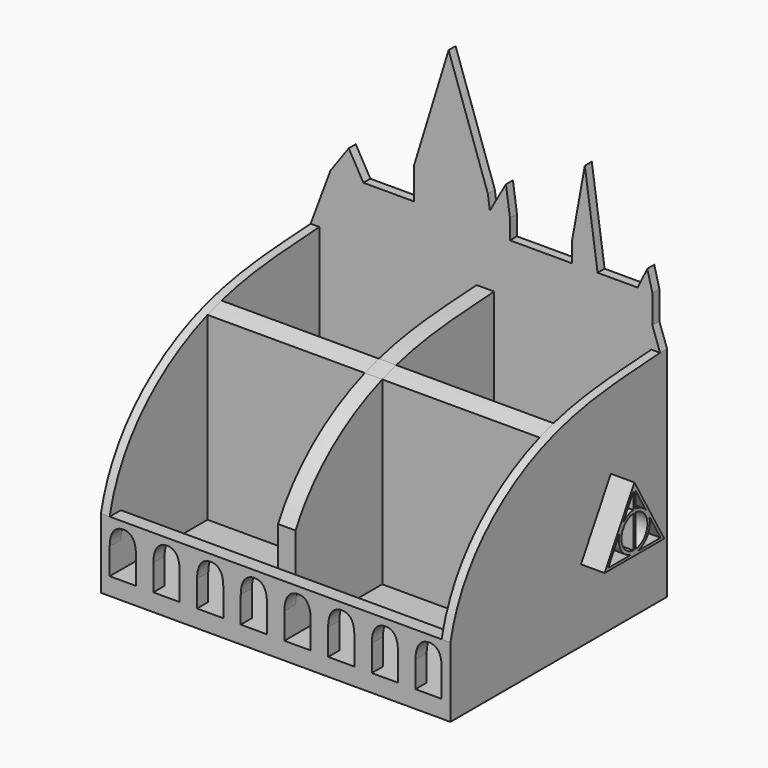
from build123d import *

# Parameters (mm, degrees)
F0_W      = 200
F0_H      = 40
F1_DEPTH  = 8
F6_W      = 200
F6_H      = 142
F7_DEPTH  = 10
F8_DEPTH  = 5
F9_DEPTH  = 5
F10_DEPTH = 5
F13_DEPTH = 90
F15_DEPTH = 90
F11_W     = 10
F11_H     = 115
F16_DEPTH = 145
F18_DEPTH = 51
F20_DEPTH = 25
F23_DEPTH = 61
F24_SCALE = 0.5
F28_DEPTH = 25


# Not quite as in the source:
# - the dataset's text gives a spline's control points without its knots; the knots are read off the source's solid


with BuildPart() as f1:
    # F0 (on Front) → F1 (new body)
    with BuildSketch(Plane.XZ):
        with Locations((-20, -45.8007189631)):
            Rectangle(F0_W, F0_H)
        with BuildLine():
            Line((-100, -55.8007189631), (-115, -55.8007189631))
            Line((-115, -55.8007189631), (-115, -40.8007189631))
            add(Edge.make_bspline(
                [(-115, -40.8007189631), (-114.9002121504, -32.0896513253), (-106.9334127401, -27.3639668916), (-99.7808481933, -32.1017122979), (-100, -40.8007189631)],
                knots=[0, 0, 0, 0, 0.50452037, 1, 1, 1, 1], degree=3))
            Line((-100, -40.8007189631), (-100, -55.8007189631))
        make_face(mode=Mode.SUBTRACT)
        with BuildLine():
            Line((-75, -55.8007189631), (-90, -55.8007189631))
            Line((-90, -55.8007189631), (-90, -40.8007189631))
            add(Edge.make_bspline(
                [(-90, -40.8007189631), (-89.9002121504, -32.0896513253), (-81.9334127401, -27.3639668916), (-74.7808481933, -32.1017122979), (-75, -40.8007189631)],
                knots=[0, 0, 0, 0, 0.50452037, 1, 1, 1, 1], degree=3))
            Line((-75, -40.8007189631), (-75, -55.8007189631))
        make_face(mode=Mode.SUBTRACT)
        with BuildLine():
            Line((-50, -55.8007189631), (-65, -55.8007189631))
            Line((-65, -55.8007189631), (-65, -40.8007189631))
            add(Edge.make_bspline(
                [(-65, -40.8007189631), (-64.9002121504, -32.0896513253), (-56.9334127401, -27.3639668916), (-49.7808481933, -32.1017122979), (-50, -40.8007189631)],
                knots=[0, 0, 0, 0, 0.50452037, 1, 1, 1, 1], degree=3))
            Line((-50, -40.8007189631), (-50, -55.8007189631))
        make_face(mode=Mode.SUBTRACT)
        with BuildLine():
            Line((-25, -55.8007189631), (-40, -55.8007189631))
            Line((-40, -55.8007189631), (-40, -40.8007189631))
            add(Edge.make_bspline(
                [(-40, -40.8007189631), (-39.9002121504, -32.0896513253), (-31.9334127401, -27.3639668916), (-24.7808481933, -32.1017122979), (-25, -40.8007189631)],
                knots=[0, 0, 0, 0, 0.50452037, 1, 1, 1, 1], degree=3))
            Line((-25, -40.8007189631), (-25, -55.8007189631))
        make_face(mode=Mode.SUBTRACT)
        with BuildLine():
            Line((0, -55.8007189631), (-15, -55.8007189631))
            Line((-15, -55.8007189631), (-15, -40.8007189631))
            add(Edge.make_bspline(
                [(-15, -40.8007189631), (-14.9002121504, -32.0896513253), (-6.9334127401, -27.3639668916), (0.2191518067, -32.1017122979), (0, -40.8007189631)],
                knots=[0, 0, 0, 0, 0.50452037, 1, 1, 1, 1], degree=3))
            Line((0, -40.8007189631), (0, -55.8007189631))
        make_face(mode=Mode.SUBTRACT)
        with BuildLine():
            Line((25, -55.8007189631), (10, -55.8007189631))
            Line((10, -55.8007189631), (10, -40.8007189631))
            add(Edge.make_bspline(
                [(10, -40.8007189631), (10.0997878496, -32.0896513253), (18.0665872599, -27.3639668916), (25.2191518067, -32.1017122979), (25, -40.8007189631)],
                knots=[0, 0, 0, 0, 0.50452037, 1, 1, 1, 1], degree=3))
            Line((25, -40.8007189631), (25, -55.8007189631))
        make_face(mode=Mode.SUBTRACT)
        with BuildLine():
            Line((50, -55.8007189631), (35, -55.8007189631))
            Line((35, -55.8007189631), (35, -40.8007189631))
            add(Edge.make_bspline(
                [(35, -40.8007189631), (35.0997878496, -32.0896513253), (43.0665872599, -27.3639668916), (50.2191518067, -32.1017122979), (50, -40.8007189631)],
                knots=[0, 0, 0, 0, 0.50452037, 1, 1, 1, 1], degree=3))
            Line((50, -40.8007189631), (50, -55.8007189631))
        make_face(mode=Mode.SUBTRACT)
        with BuildLine():
            Line((75, -55.8007189631), (60, -55.8007189631))
            Line((60, -55.8007189631), (60, -40.8007189631))
            add(Edge.make_bspline(
                [(60, -40.8007189631), (60.0997878496, -32.0896513253), (68.0665872599, -27.3639668916), (75.2191518067, -32.1017122979), (75, -40.8007189631)],
                knots=[0, 0, 0, 0, 0.50452037, 1, 1, 1, 1], degree=3))
            Line((75, -40.8007189631), (75, -55.8007189631))
        make_face(mode=Mode.SUBTRACT)
    extrude(amount=F1_DEPTH)

    # F6 (on face) → F7 (join)
    with BuildSketch(Plane(origin=(0, 0, -65.8007189631), x_dir=(1, 0, 0), z_dir=(0, 0, -1))):
        with Locations((-20, -71)):
            Rectangle(F6_W, F6_H)
    extrude(amount=-F7_DEPTH)

    # F2 (on face) → F8 (join)
    with BuildSketch(Plane.YZ.offset(80)):
        with BuildLine():
            Line((0, -25.8007189631), (0, -65.8007189631))
            Line((0, -65.8007189631), (142, -65.8007189631))
            Line((142, -65.8007189631), (142, 59.1992810369))
            add(Edge.make_bspline(
                [(142, 59.1992810369), (115.2555122972, 57.2821311653), (55.7364718353, 56.513611212), (0, 11.2629952783), (-8, -25.8007189631)],
                knots=[0, 0, 0, 0, 0.4803328579, 1, 1, 1, 1], degree=3))
            Line((-8, -25.8007189631), (0, -25.8007189631))
        make_face()
    extrude(amount=-F8_DEPTH)

    # F5 (on face) → F9 (join)
    with BuildSketch(Plane(origin=(-120, 0, 0), x_dir=(0, -1, 0), z_dir=(-1, 0, 0))):
        with BuildLine():
            add(Edge.make_bspline(
                [(-142, 59.1992810369), (-115.2555122972, 57.2821311653), (-55.7364718353, 56.513611212), (0, 11.2629952783), (8, -25.8007189631)],
                knots=[0, 0, 0, 0, 0.4803328579, 1, 1, 1, 1], degree=3))
            Line((-142, 59.1992810369), (-142, -65.8007189631))
            Line((-142, -65.8007189631), (0, -65.8007189631))
            Line((0, -65.8007189631), (0, -25.8007189631))
            Line((0, -25.8007189631), (8, -25.8007189631))
        make_face()
    extrude(amount=-F9_DEPTH)

    # F4 (on offset) → F10 (join)
    with BuildSketch(Plane(origin=(0, 142, 0), x_dir=(-1, 0, 0), z_dir=(0, 1, 0))):
        Polygon((-75.6055936217, 71.6397762299), (-80, 59.1992810369), (-80, -65.8007189631), (120, -65.8007189631), (120, 59.1992810369), (108.6526662111, 89.6646231413), (98.1675684452, 104.3437644839), (89.7794961929, 89.6646231413), (60.8406178653, 89.6646231413), (60.8406178653, 107.6989993453), (41.0309545696, 172.3506748676), (18.570561702, 107.3117282984), (17.4182727933, 99.1869866848), (8.212401149, 115.4364699119), (5.9078233317, 99.1869866848), (5.9078233317, 87.9176706076), (-29.613243416, 87.9176706076), (-29.613243416, 99.1869866848), (-36.9290038943, 139.5011246204), (-44.2448109388, 87.9176706076), (-67.2579482198, 87.9176706076), (-72.6839154959, 99.1869866848), (-75.6055936217, 87.9176706076), align=None)
    extrude(amount=F10_DEPTH)

    # F12 (on face) → F13 (join)
    with BuildSketch(Plane.YZ.offset(-115)):
        with BuildLine():
            Line((62, 47.4087703187), (62, -55.8007189631))
            Line((62, -55.8007189631), (72, -55.8007189631))
            Line((72, -55.8007189631), (72, 50.5592355273))
            add(Edge.make_bspline(
                [(72, 50.5592355273), (68.6586994693, 49.6363485793), (65.3238142049, 48.5929393736), (62, 47.4087703187)],
                knots=[0.4052571345, 0.4052571345, 0.4052571345, 0.4052571345, 0.4627350394, 0.4627350394, 0.4627350394, 0.4627350394], degree=3))
        make_face()
    extrude(amount=F13_DEPTH)

    # F14 (on face) → F15 (join)
    with BuildSketch(Plane(origin=(75, 0, 0), x_dir=(0, -1, 0), z_dir=(-1, 0, 0))):
        with BuildLine():
            Line((-72, 50.5592355273), (-72, -55.8007189631))
            Line((-72, -55.8007189631), (-62, -55.8007189631))
            Line((-62, -55.8007189631), (-62, 47.4087703187))
            add(Edge.make_bspline(
                [(-72, 50.5592355273), (-68.6586994693, 49.6363485793), (-65.3238142049, 48.5929393736), (-62, 47.4087703187)],
                knots=[0.4052571345, 0.4052571345, 0.4052571345, 0.4052571345, 0.4627350394, 0.4627350394, 0.4627350394, 0.4627350394], degree=3))
        make_face()
    extrude(amount=F15_DEPTH)

    # F11 (on face) → F16 (join)
    with BuildSketch(Plane.XZ.offset(-142)):
        with Locations((-20, 1.6992810369)):
            Rectangle(F11_W, F11_H)
    extrude(amount=F16_DEPTH)

    # F17 (on face) → F18 (cut)
    with BuildSketch(Plane.YZ.offset(-15)):
        with BuildLine():
            add(Edge.make_bspline(
                [(142, 59.1992810369), (119.4356588951, 57.5817804838), (95.5583722327, 57.0661971279), (72, 50.5592355273)],
                knots=[0, 0, 0, 0, 0.4052571345, 0.4052571345, 0.4052571345, 0.4052571345], degree=3))
            Line((142, 59.1992810369), (-3, 59.1992810369))
            Line((-3, 59.1992810369), (-3, -9.9070407138))
            add(Edge.make_bspline(
                [(62, 47.4087703187), (60.982358885, 47.0462172266), (34.4860149895, 37.2528805245), (8.785415014, 18.1017869852), (-3, -9.9070407138)],
                knots=[0.4627350394, 0.4627350394, 0.4627350394, 0.4627350394, 0.4803328579, 0.9213975632, 0.9213975632, 0.9213975632, 0.9213975632], degree=3))
            add(Edge.make_bspline(
                [(72, 50.5592355273), (68.6586994693, 49.6363485793), (65.3238142049, 48.5929393736), (62, 47.4087703187)],
                knots=[0.4052571345, 0.4052571345, 0.4052571345, 0.4052571345, 0.4627350394, 0.4627350394, 0.4627350394, 0.4627350394], degree=3))
        make_face()
    extrude(amount=-F18_DEPTH, mode=Mode.SUBTRACT)

    # F19 (on face) → F20 (cut)
    with BuildSketch(Plane.YZ.offset(-15)):
        with BuildLine():
            Line((-3, -25.8007189631), (0, -25.8007189631))
            Line((0, -25.8007189631), (0, -3.5044075334))
            add(Edge.make_bspline(
                [(0, -3.5044075334), (-1.0753491863, -5.5801208083), (-2.0772996861, -7.714181652), (-3, -9.9070407138)],
                knots=[0.8868658525, 0.8868658525, 0.8868658525, 0.8868658525, 0.9213975632, 0.9213975632, 0.9213975632, 0.9213975632], degree=3))
            Line((-3, -9.9070407212), (-3, -25.8007189631))
        make_face()
    extrude(amount=-F20_DEPTH, mode=Mode.SUBTRACT)

    # F27 (on offset) → F28 (cut)
    with BuildSketch(Plane.YZ.offset(80)):
        with BuildLine():
            Line((96.2274455769, -8.6646838435), (88.0223984364, -22.8762423694))
            Line((88.0223984364, -22.8762423694), (104.4324927174, -22.8762423694))
            ThreePointArc((104.4324927174, -22.8762423694), (97.1808920854, -17.5885835957), (96.2274455769, -8.6646838435))
        make_face()
        with BuildLine():
            Line((106.0223984364, -21.3460336088), (106.0223984364, -2.7558160353))
            ThreePointArc((106.0223984364, -2.7558160353), (97.4470808891, -12.0509248221), (106.0223984364, -21.3460336088))
        make_face()
        with BuildLine():
            Line((107.5223984364, -2.7558160353), (107.5223984364, -21.3460336088))
            ThreePointArc((107.5223984364, -21.3460336088), (116.0977159837, -12.0509248221), (107.5223984364, -2.7558160353))
        make_face()
        with BuildLine():
            ThreePointArc((107.5397189444, -1.0022200106), (111.6080162168, -2.0870169815), (114.9774455769, -4.6118482533))
            Line((114.9774455769, -4.6118482533), (107.5223984364, 8.3006721669))
            Line((107.5223984364, 8.3006721669), (107.5223984364, -1.0010171202))
            Line((107.5223984364, -1.0010171202), (107.5397189444, -1.0022200106))
        make_face()
        with BuildLine():
            Line((106.0223984364, 8.3006721669), (98.5673512959, -4.6118482533))
            ThreePointArc((98.5673512959, -4.6118482533), (101.936780656, -2.0870169815), (106.0050779283, -1.0022200106))
            Line((106.0050779283, -1.0022200106), (106.0223984364, -1.0010171202))
            Line((106.0223984364, -1.0010171202), (106.0223984364, 8.3006721669))
        make_face()
        with BuildLine():
            ThreePointArc((117.3173512959, -8.6646838435), (116.3639047873, -17.5885835957), (109.1123041553, -22.8762423694))
            Line((109.1123041553, -22.8762423694), (125.5223984364, -22.8762423694))
            Line((125.5223984364, -22.8762423694), (117.3173512959, -8.6646838435))
        make_face()
    extrude(amount=-F28_DEPTH, mode=Mode.SUBTRACT)


with BuildPart() as f23:
    # F22 (on offset) → F23 (new body)
    with BuildSketch(Plane.YZ.offset(80)):
        Polygon((65.5447968727, 25.1994205451), (22.84864445, -48.7524847387), (108.2409492955, -48.7524847387), align=None)
        with BuildLine():
            Line((60.8649854348, -45.7524847387), (28.0447968727, -45.7524847387))
            Line((28.0447968727, -45.7524847387), (44.4548911538, -17.329367687))
            ThreePointArc((44.4548911538, -17.329367687), (46.3617841709, -35.1771671914), (60.8649854348, -45.7524847387))
        make_face(mode=Mode.SUBTRACT)
        with BuildLine():
            ThreePointArc((64.0447968727, -42.6920672177), (46.8941617781, -24.1018496441), (64.0447968727, -5.5116320706))
            Line((64.0447968727, -5.5116320706), (64.0447968727, -42.6920672177))
        make_face(mode=Mode.SUBTRACT)
        with BuildLine():
            Line((103.0447968727, -45.7524847387), (70.2246083107, -45.7524847387))
            ThreePointArc((70.2246083107, -45.7524847387), (84.7278095746, -35.1771671914), (86.6347025917, -17.329367687))
            Line((86.6347025917, -17.329367687), (103.0447968727, -45.7524847387))
        make_face(mode=Mode.SUBTRACT)
        with BuildLine():
            Line((67.0447968727, -42.6920672177), (67.0447968727, -5.5116320706))
            ThreePointArc((67.0447968727, -5.5116320706), (84.1954319674, -24.1018496441), (67.0447968727, -42.6920672177))
        make_face(mode=Mode.SUBTRACT)
        with BuildLine():
            Line((49.1347025917, -9.2236965066), (64.0447968727, 16.6013443337))
            Line((64.0447968727, 16.6013443337), (64.0447968727, -2.0020342403))
            Line((64.0447968727, -2.0020342403), (64.0101558566, -2.0044400211))
            ThreePointArc((64.0101558566, -2.0044400211), (55.8735613119, -4.174033963), (49.1347025917, -9.2236965066))
        make_face(mode=Mode.SUBTRACT)
        with BuildLine():
            Line((67.0447968727, -2.0020342403), (67.0447968727, 16.6013443337))
            Line((67.0447968727, 16.6013443337), (81.9548911538, -9.2236965066))
            ThreePointArc((81.9548911538, -9.2236965066), (75.2160324335, -4.174033963), (67.0794378889, -2.0044400211))
            Line((67.0794378889, -2.0044400211), (67.0447968727, -2.0020342403))
        make_face(mode=Mode.SUBTRACT)
    extrude(amount=F23_DEPTH)


with BuildPart() as f23_1:
    # F24: moved
    add(f23.part.scale(F24_SCALE))


with BuildPart() as f23_2:
    # F25: moved
    add(f23_1.part.moved(Location((23, 74, 0))))


solid = Compound([f1.part, f23_2.part])
